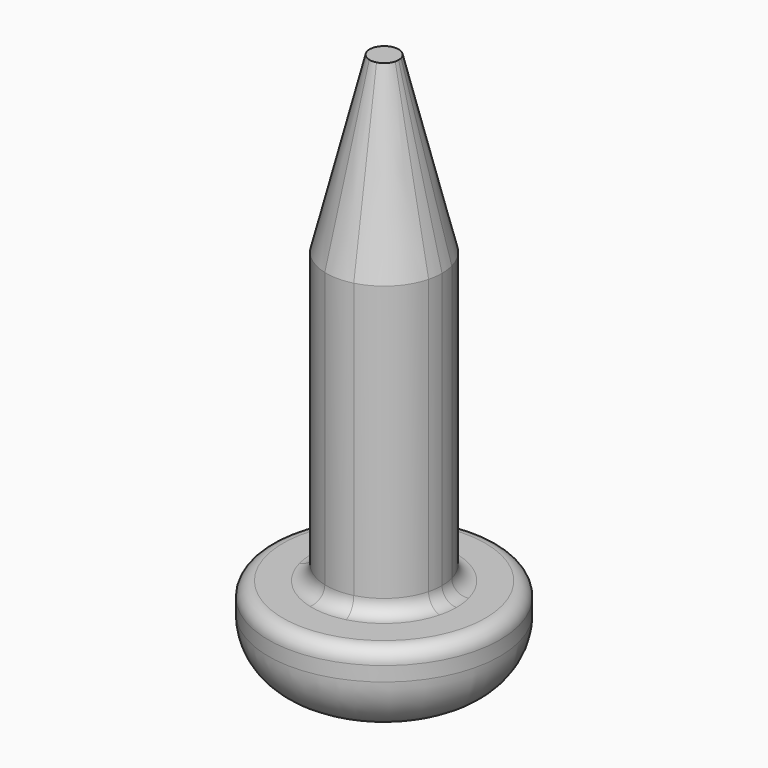
from build123d import *

# Parameters (mm, degrees)
F0_R     = 2
F1_DEPTH = 1
F2_START = 1
F0_W     = 0.5
F0_H     = 0.5
F2_DEPTH = 0.5
F3_START = 1.5
F3_DEPTH = 8
F4_SIZE2 = 3
F4_SIZE  = 0.75
F6_R     = 0.25


# Not quite as in the source:
# - a fillet or chamfer that OpenCascade refuses, or shapes differently, is made with other operations: its cross-section is extruded or revolved along the edge and cut away or added


with BuildPart() as f1:
    # F0 (on Top) → F1 (new body)
    with BuildSketch(Plane.XY):
        Circle(F0_R)
        with BuildLine():
            ThreePointArc((0.25, 0.9682458366), (0.7071067812, 0.7071067812), (0.9682458366, 0.25))
            Line((0.9682458366, 0.25), (1.25, 0.25))
            Line((1.25, 0.25), (1.25, -0.25))
            Line((1.25, -0.25), (0.9682458366, -0.25))
            ThreePointArc((0.9682458366, -0.25), (0.7071067812, -0.7071067812), (0.25, -0.9682458366))
            Line((0.25, -0.9682458366), (0.25, -1.25))
            Line((0.25, -1.25), (-0.25, -1.25))
            Line((-0.25, -1.25), (-0.25, -0.9682458366))
            ThreePointArc((-0.25, -0.9682458366), (-0.7071067812, -0.7071067812), (-0.9682458366, -0.25))
            Line((-0.9682458366, -0.25), (-1.25, -0.25))
            Line((-1.25, -0.25), (-1.25, 0.25))
            Line((-1.25, 0.25), (-0.9682458366, 0.25))
            ThreePointArc((-0.9682458366, 0.25), (-0.7071067812, 0.7071067812), (-0.25, 0.9682458366))
            Line((-0.25, 0.9682458366), (-0.25, 1.25))
            Line((-0.25, 1.25), (0.25, 1.25))
            Line((0.25, 1.25), (0.25, 0.9682458366))
        make_face(mode=Mode.SUBTRACT)
        with BuildLine():
            Line((-0.25, 0.25), (-0.25, 0.9682458366))
            ThreePointArc((-0.25, 0.9682458366), (-0.7071067812, 0.7071067812), (-0.9682458366, 0.25))
            Line((-0.9682458366, 0.25), (-0.25, 0.25))
        make_face()
        with BuildLine():
            ThreePointArc((-0.9682458366, -0.25), (-0.7071067812, -0.7071067812), (-0.25, -0.9682458366))
            Line((-0.25, -0.9682458366), (-0.25, -0.25))
            Line((-0.25, -0.25), (-0.9682458366, -0.25))
        make_face()
        with BuildLine():
            ThreePointArc((0.25, -0.9682458366), (0.7071067812, -0.7071067812), (0.9682458366, -0.25))
            Line((0.9682458366, -0.25), (0.25, -0.25))
            Line((0.25, -0.25), (0.25, -0.9682458366))
        make_face()
        with BuildLine():
            Line((0.25, 0.25), (0.9682458366, 0.25))
            ThreePointArc((0.9682458366, 0.25), (0.7071067812, 0.7071067812), (0.25, 0.9682458366))
            Line((0.25, 0.9682458366), (0.25, 0.25))
        make_face()
    extrude(amount=F1_DEPTH)

    # F0 (on Top) → F2 (join)
    with BuildSketch(Plane.XY.offset(F2_START)):
        Circle(F0_R)
        with BuildLine():
            ThreePointArc((0.25, 0.9682458366), (0.7071067812, 0.7071067812), (0.9682458366, 0.25))
            Line((0.9682458366, 0.25), (1.25, 0.25))
            Line((1.25, 0.25), (1.25, -0.25))
            Line((1.25, -0.25), (0.9682458366, -0.25))
            ThreePointArc((0.9682458366, -0.25), (0.7071067812, -0.7071067812), (0.25, -0.9682458366))
            Line((0.25, -0.9682458366), (0.25, -1.25))
            Line((0.25, -1.25), (-0.25, -1.25))
            Line((-0.25, -1.25), (-0.25, -0.9682458366))
            ThreePointArc((-0.25, -0.9682458366), (-0.7071067812, -0.7071067812), (-0.9682458366, -0.25))
            Line((-0.9682458366, -0.25), (-1.25, -0.25))
            Line((-1.25, -0.25), (-1.25, 0.25))
            Line((-1.25, 0.25), (-0.9682458366, 0.25))
            ThreePointArc((-0.9682458366, 0.25), (-0.7071067812, 0.7071067812), (-0.25, 0.9682458366))
            Line((-0.25, 0.9682458366), (-0.25, 1.25))
            Line((-0.25, 1.25), (0.25, 1.25))
            Line((0.25, 1.25), (0.25, 0.9682458366))
        make_face(mode=Mode.SUBTRACT)
        with BuildLine():
            Line((0.25, 0.25), (0.25, 0.9682458366))
            ThreePointArc((0.25, 0.9682458366), (0, 1), (-0.25, 0.9682458366))
            Line((-0.25, 0.9682458366), (-0.25, 0.25))
            Line((-0.25, 0.25), (0.25, 0.25))
        make_face()
        with BuildLine():
            ThreePointArc((-0.25, -0.9682458366), (0, -1), (0.25, -0.9682458366))
            Line((0.25, -0.9682458366), (0.25, -0.25))
            Line((0.25, -0.25), (-0.25, -0.25))
            Line((-0.25, -0.25), (-0.25, -0.9682458366))
        make_face()
        with BuildLine():
            ThreePointArc((0.9682458366, -0.25), (0.9920296963, -0.1260042925), (1, 0))
            ThreePointArc((1, 0), (0.9920296963, 0.1260042925), (0.9682458366, 0.25))
            Line((0.9682458366, 0.25), (0.25, 0.25))
            Line((0.25, 0.25), (0.25, -0.25))
            Line((0.25, -0.25), (0.9682458366, -0.25))
        make_face()
        with BuildLine():
            Line((-0.25, -0.25), (-0.25, 0.25))
            Line((-0.25, 0.25), (-0.9682458366, 0.25))
            ThreePointArc((-0.9682458366, 0.25), (-1, 0), (-0.9682458366, -0.25))
            Line((-0.9682458366, -0.25), (-0.25, -0.25))
        make_face()
        with BuildLine():
            ThreePointArc((-0.9682458366, -0.25), (-0.7071067812, -0.7071067812), (-0.25, -0.9682458366))
            Line((-0.25, -0.9682458366), (-0.25, -0.25))
            Line((-0.25, -0.25), (-0.9682458366, -0.25))
        make_face()
        with BuildLine():
            ThreePointArc((0.25, -0.9682458366), (0.7071067812, -0.7071067812), (0.9682458366, -0.25))
            Line((0.9682458366, -0.25), (0.25, -0.25))
            Line((0.25, -0.25), (0.25, -0.9682458366))
        make_face()
        with BuildLine():
            Line((0.25, 0.25), (0.9682458366, 0.25))
            ThreePointArc((0.9682458366, 0.25), (0.7071067812, 0.7071067812), (0.25, 0.9682458366))
            Line((0.25, 0.9682458366), (0.25, 0.25))
        make_face()
        with BuildLine():
            Line((-0.25, 0.25), (-0.25, 0.9682458366))
            ThreePointArc((-0.25, 0.9682458366), (-0.7071067812, 0.7071067812), (-0.9682458366, 0.25))
            Line((-0.9682458366, 0.25), (-0.25, 0.25))
        make_face()
        Rectangle(F0_W, F0_H)
        with BuildLine():
            ThreePointArc((-0.9682458366, -0.25), (-1, 0), (-0.9682458366, 0.25))
            Line((-0.9682458366, 0.25), (-1.25, 0.25))
            Line((-1.25, 0.25), (-1.25, -0.25))
            Line((-1.25, -0.25), (-0.9682458366, -0.25))
        make_face()
        with BuildLine():
            ThreePointArc((0.9682458366, 0.25), (0.9920296963, 0.1260042925), (1, 0))
            ThreePointArc((1, 0), (0.9920296963, -0.1260042925), (0.9682458366, -0.25))
            Line((0.9682458366, -0.25), (1.25, -0.25))
            Line((1.25, -0.25), (1.25, 0.25))
            Line((1.25, 0.25), (0.9682458366, 0.25))
        make_face()
        with BuildLine():
            ThreePointArc((-0.25, 0.9682458366), (0, 1), (0.25, 0.9682458366))
            Line((0.25, 0.9682458366), (0.25, 1.25))
            Line((0.25, 1.25), (-0.25, 1.25))
            Line((-0.25, 1.25), (-0.25, 0.9682458366))
        make_face()
        with BuildLine():
            Line((0.25, -1.25), (0.25, -0.9682458366))
            ThreePointArc((0.25, -0.9682458366), (0, -1), (-0.25, -0.9682458366))
            Line((-0.25, -0.9682458366), (-0.25, -1.25))
            Line((-0.25, -1.25), (0.25, -1.25))
        make_face()
    extrude(amount=F2_DEPTH)

    # F0 (on Top) → F3 (join)
    with BuildSketch(Plane.XY.offset(F3_START)):
        with BuildLine():
            ThreePointArc((-0.9682458366, -0.25), (-0.7071067812, -0.7071067812), (-0.25, -0.9682458366))
            Line((-0.25, -0.9682458366), (-0.25, -0.25))
            Line((-0.25, -0.25), (-0.9682458366, -0.25))
        make_face()
        with BuildLine():
            Line((-0.25, -0.25), (-0.25, 0.25))
            Line((-0.25, 0.25), (-0.9682458366, 0.25))
            ThreePointArc((-0.9682458366, 0.25), (-1, 0), (-0.9682458366, -0.25))
            Line((-0.9682458366, -0.25), (-0.25, -0.25))
        make_face()
        with BuildLine():
            Line((-0.25, 0.25), (-0.25, 0.9682458366))
            ThreePointArc((-0.25, 0.9682458366), (-0.7071067812, 0.7071067812), (-0.9682458366, 0.25))
            Line((-0.9682458366, 0.25), (-0.25, 0.25))
        make_face()
        with BuildLine():
            Line((0.25, 0.25), (0.25, 0.9682458366))
            ThreePointArc((0.25, 0.9682458366), (0, 1), (-0.25, 0.9682458366))
            Line((-0.25, 0.9682458366), (-0.25, 0.25))
            Line((-0.25, 0.25), (0.25, 0.25))
        make_face()
        with BuildLine():
            Line((0.25, 0.25), (0.9682458366, 0.25))
            ThreePointArc((0.9682458366, 0.25), (0.7071067812, 0.7071067812), (0.25, 0.9682458366))
            Line((0.25, 0.9682458366), (0.25, 0.25))
        make_face()
        with BuildLine():
            ThreePointArc((0.9682458366, -0.25), (0.9920296963, -0.1260042925), (1, 0))
            ThreePointArc((1, 0), (0.9920296963, 0.1260042925), (0.9682458366, 0.25))
            Line((0.9682458366, 0.25), (0.25, 0.25))
            Line((0.25, 0.25), (0.25, -0.25))
            Line((0.25, -0.25), (0.9682458366, -0.25))
        make_face()
        with BuildLine():
            ThreePointArc((-0.25, -0.9682458366), (0, -1), (0.25, -0.9682458366))
            Line((0.25, -0.9682458366), (0.25, -0.25))
            Line((0.25, -0.25), (-0.25, -0.25))
            Line((-0.25, -0.25), (-0.25, -0.9682458366))
        make_face()
        with BuildLine():
            ThreePointArc((0.25, -0.9682458366), (0.7071067812, -0.7071067812), (0.9682458366, -0.25))
            Line((0.9682458366, -0.25), (0.25, -0.25))
            Line((0.25, -0.25), (0.25, -0.9682458366))
        make_face()
        Rectangle(F0_W, F0_H)
    extrude(amount=F3_DEPTH)

    # F4
    f4_edges = [f1.edges().sort_by_distance(p)[0] for p in [
        (-0.25, 0.968246, 9.5),
    ]]
    f4_side = f1.faces().sort_by_distance((0, 0, 9.5))[0]
    chamfer(f4_edges, length=F4_SIZE, length2=F4_SIZE2, reference=f4_side)

    # F5: fillet of radius 1 on 1 edges, made by hand

    # F5_s1 → F5_t2 (revolve, cut)
    with BuildSketch(Plane.XZ):
        with BuildLine():
            ThreePointArc((2, 1), (1.7071067812, 0.2928932188), (1, 0))
            Line((1, 0), (2, 0))
            Line((2, 0), (2, 1))
        make_face()
    revolve(axis=Axis((0, 0, 0), (0, 0, 1)), mode=Mode.SUBTRACT)

    # F6
    f6_edges = [f1.edges().sort_by_distance(p)[0] for p in [
        (-2, 0, 1.5),
        (-0.25, 0.968246, 1.5),
    ]]
    fillet(f6_edges, radius=F6_R)


solid = f1.part
